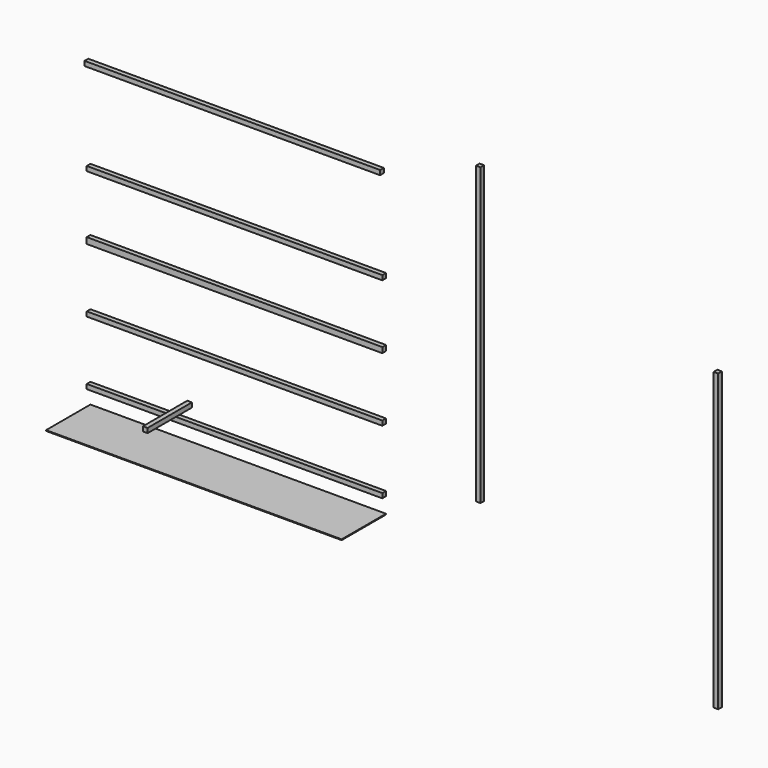
from build123d import *

# Parameters (mm, degrees)
F0_W      = 2438.4
F0_H      = 38.1
F1_DEPTH  = 38.1
F0_W_2    = 38.1
F0_H_2    = 2438.4
F2_DEPTH  = 38.1
F3_DEPTH  = 38.1
F4_DEPTH  = 38.1
F5_DEPTH  = 38.1
F6_DEPTH  = 38.1
F7_E6_W   = 2438.4
F7_E6_H   = 457.2
F8_DEPTH  = 6.35
F9_DEPTH  = 38.1
F10_W     = 457.2
F10_H     = 38.1
F11_DEPTH = 38.1


with BuildPart() as f1:
    # F0 (on Front) → F1 (new body)
    with BuildSketch(Plane.XZ):
        with Locations((121.9220010757, 779.5966842651)):
            Rectangle(F0_W, F0_H)
    extrude(amount=F1_DEPTH)


with BuildPart() as f2:
    # F0 (on Front) → F2 (new body)
    with BuildSketch(Plane.XZ):
        with Locations((2150.5049446106, -131.9238098145)):
            Rectangle(F0_W_2, F0_H_2)
    extrude(amount=F2_DEPTH)


with BuildPart() as f3:
    # F0 (on Front) → F3 (new body)
    with BuildSketch(Plane.XZ):
        with Locations((140.006583941, -1560.925090957)):
            Rectangle(F0_W, F0_H)
    extrude(amount=F3_DEPTH)


with BuildPart() as f4:
    # F0 (on Front) → F4 (new body)
    with BuildSketch(Plane.XZ):
        with Locations((140.006583941, -1033.875090957)):
            Rectangle(F0_W, F0_H)
    extrude(amount=F4_DEPTH)


with BuildPart() as f5:
    # F0 (on Front) → F5 (new body)
    with BuildSketch(Plane.XZ):
        Polygon((1359.206583941, 7.0199789283), (1359.206583941, 41.2889796493), (-1079.193416059, 41.2889796493), (-1079.193416059, 13.3699789283), (-1079.193416059, 3.1889796493), (1359.206583941, 3.1889796493), align=None)
    extrude(amount=F5_DEPTH)


with BuildPart() as f6:
    # F0 (on Front) → F6 (new body)
    with BuildSketch(Plane.XZ):
        Polygon((1359.206583941, -525.875090957), (1359.206583941, -481.425090957), (-1079.193416059, -475.5800210717), (-1079.193416059, -525.875090957), align=None)
    extrude(amount=F6_DEPTH)


with BuildPart() as f8:
    # F7_E6 (on explicit) → F8 (new body)
    with BuildSketch(Plane(origin=(-1079.193416059, 0, -1713.325090957), x_dir=(1, 0, 0), z_dir=(0, 0, -1))):
        with Locations((1219.2, 228.6)):
            Rectangle(F7_E6_W, F7_E6_H)
    extrude(amount=-F8_DEPTH)


with BuildPart() as f9:
    # F0 (on Front) → F9 (new body)
    with BuildSketch(Plane.XZ):
        with Locations((4111.2189292908, -991.5800094604)):
            Rectangle(F0_W_2, F0_H_2)
    extrude(amount=F9_DEPTH)


with BuildPart() as f11:
    # F10 (on Right) → F11 (new body)
    with BuildSketch(Plane.YZ):
        with Locations((-578.8760185242, -1204.6841109155)):
            Rectangle(F10_W, F10_H)
    extrude(amount=F11_DEPTH)


solid = Compound([f1.part, f2.part, f3.part, f4.part, f5.part, f6.part, f8.part, f9.part, f11.part])
